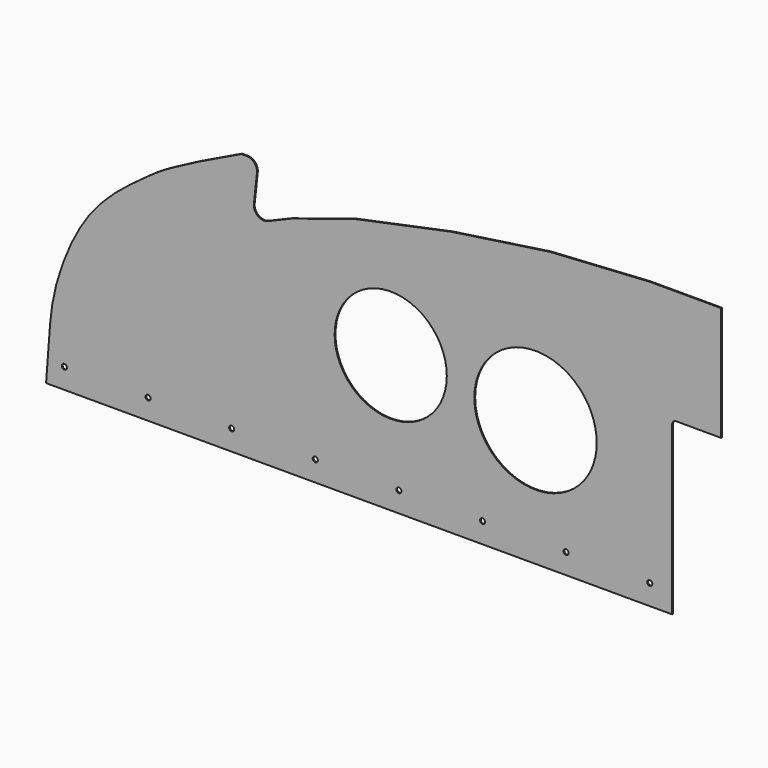
from build123d import *

# Parameters (mm, degrees)
F0_R        = 1.25
F1_DEPTH    = 0.5
F2_R        = 5
F3_T1_DEPTH = 74.0375335511
F3_T3_DEPTH = 9.1893951821
F3_T5_DEPTH = 38.8426126869
F3_T7_DEPTH = 73.4476683762
F4_R        = 100
F5_R        = 5
F6_R        = 2


# Not quite as in the source:
# - a fillet or chamfer that OpenCascade refuses, or shapes differently, is made with other operations: its cross-section is extruded or revolved along the edge and cut away or added


with BuildPart() as f1:
    # F0 (on Front) → F1 (new body)
    with BuildSketch(Plane.XZ):
        with BuildLine():
            Line((-65, 0), (-24, 0))
            Line((-24, 0), (-24, 84))
            Line((-24, 84), (0, 84))
            Line((0, 84), (0, 140))
            Line((0, 140), (-35, 140))
            Line((-35, 140), (-84, 137))
            Line((-84, 137), (-132, 130))
            Line((-132, 130), (-180, 120))
            Line((-180, 120), (-211, 110))
            Line((-211, 110), (-230, 102))
            Line((-230, 102), (-227, 130))
            Line((-227, 130), (-235.2838218212, 130))
            Line((-235.2838218212, 130), (-256, 120))
            Line((-256, 120), (-275, 110))
            Line((-275, 110), (-302, 90))
            Line((-302, 90), (-311, 78))
            Line((-311, 78), (-311, 0))
            Line((-311, 0), (-270, 0))
            Line((-270, 0), (-229, 0))
            Line((-229, 0), (-188, 0))
            Line((-188, 0), (-188, 58.0417635664))
            ThreePointArc((-188, 58.0417635664), (-189.5, 67), (-188, 75.9582364336))
            ThreePointArc((-188, 75.9582364336), (-157.4585244689, 94.1224077102), (-134.5, 67))
            ThreePointArc((-134.5, 67), (-137.8261504927, 53.8898893979), (-147, 43.9511388568))
            Line((-147, 43.9511388568), (-147, 0))
            Line((-147, 0), (-106, 0))
            Line((-106, 0), (-106, 36.0192378865))
            ThreePointArc((-106, 36.0192378865), (-112.1995806787, 83.2268174498), (-65, 76.9666295471))
            ThreePointArc((-65, 76.9666295471), (-62.0172465076, 69.7459666924), (-61, 62))
            ThreePointArc((-61, 62), (-62.0172465076, 54.2540333076), (-65, 47.0333704529))
            Line((-65, 47.0333704529), (-65, 0))
        make_face()
        with Locations((-281, 10)):
            Circle(F0_R, mode=Mode.SUBTRACT)
        with Locations((-240, 10)):
            Circle(F0_R, mode=Mode.SUBTRACT)
        with Locations((-199, 10)):
            Circle(F0_R, mode=Mode.SUBTRACT)
        with Locations((-117, 10)):
            Circle(F0_R, mode=Mode.SUBTRACT)
        with Locations((-35, 10)):
            Circle(F0_R, mode=Mode.SUBTRACT)
        Polygon((-331, 0), (-311, 0), (-311, 78), (-317, 70), (-328, 40), align=None)
        with Locations((-322, 10)):
            Circle(F0_R, mode=Mode.SUBTRACT)
        with BuildLine():
            Line((-188, 0), (-147, 0))
            Line((-147, 0), (-147, 43.9511388568))
            ThreePointArc((-147, 43.9511388568), (-170.9379206853, 40.9930091356), (-188, 58.0417635664))
            Line((-188, 58.0417635664), (-188, 0))
        make_face()
        with Locations((-158, 10)):
            Circle(F0_R, mode=Mode.SUBTRACT)
        with BuildLine():
            Line((-106, 0), (-65, 0))
            Line((-65, 0), (-65, 47.0333704529))
            ThreePointArc((-65, 47.0333704529), (-83.2168271863, 33.0272158578), (-106, 36.0192378865))
            Line((-106, 36.0192378865), (-106, 0))
        make_face()
        with Locations((-76, 10)):
            Circle(F0_R, mode=Mode.SUBTRACT)
    extrude(amount=F1_DEPTH)

    # F2
    f2_edges = [f1.edges().sort_by_distance(p)[0] for p in [
        (-230, -0.25, 102),
    ]]
    fillet(f2_edges, radius=F2_R)

    # F3: fillet of radius 100 on 4 edges, made by hand

    # F3_s2 → F3_t1 (cut)
    with BuildSketch(Plane.XZ.offset(-36.7687667756)):
        with BuildLine():
            ThreePointArc((-308.1754959739, 81.7660053682), (-316.0546249868, 69.4866370062), (-322.0631275625, 56.191470284))
            Line((-322.0631275625, 56.191470284), (-317, 70))
            Line((-317, 70), (-308.1754959739, 81.7660053682))
        make_face()
    extrude(amount=F3_T1_DEPTH, mode=Mode.SUBTRACT)

    # F3_s4 → F3_t3 (cut)
    with BuildSketch(Plane.XZ.offset(-4.3446975911)):
        with BuildLine():
            ThreePointArc((-254.4349231681, 120.7554853112), (-255.9932004856, 119.9865175696), (-257.5378808276, 119.1905890381))
            Line((-257.5378808276, 119.1905890381), (-256, 120))
            Line((-256, 120), (-254.4349231681, 120.7554853112))
        make_face()
    extrude(amount=F3_T3_DEPTH, mode=Mode.SUBTRACT)

    # F3_s6 → F3_t5 (cut)
    with BuildSketch(Plane.XZ.offset(-19.1713063434)):
        with BuildLine():
            ThreePointArc((-268.2139846679, 113.5715870169), (-274.8437916361, 109.7514039115), (-281.1620964472, 105.4354841132))
            Line((-281.1620964472, 105.4354841132), (-275, 110))
            Line((-275, 110), (-268.2139846679, 113.5715870169))
        make_face()
    extrude(amount=F3_T5_DEPTH, mode=Mode.SUBTRACT)

    # F3_s8 → F3_t7 (cut)
    with BuildSketch(Plane.XZ.offset(-36.4738341881)):
        with BuildLine():
            ThreePointArc((-290.2764752677, 98.6840923943), (-301.2536395134, 89.2491836695), (-310.7537202051, 78.3283730598))
            Line((-310.7537202051, 78.3283730598), (-302, 90))
            Line((-302, 90), (-290.2764752677, 98.6840923943))
        make_face()
    extrude(amount=F3_T7_DEPTH, mode=Mode.SUBTRACT)

    # F4
    f4_edges = [f1.edges().sort_by_distance(p)[0] for p in [
        (-328, -0.25, 40),
    ]]
    fillet(f4_edges, radius=F4_R)

    # F5
    f5_edges = [f1.edges().sort_by_distance(p)[0] for p in [
        (-227, -0.25, 130),
    ]]
    fillet(f5_edges, radius=F5_R)

    # F6
    f6_edges = [f1.edges().sort_by_distance(p)[0] for p in [
        (-24, -0.25, 84),
    ]]
    fillet(f6_edges, radius=F6_R)


solid = f1.part
